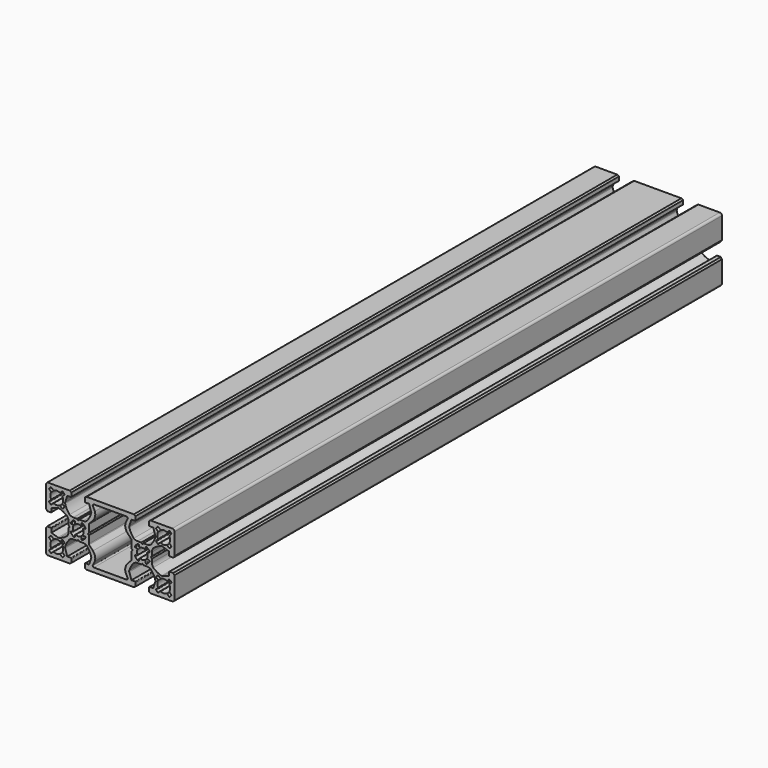
from build123d import *

# Parameters (mm, degrees)
F1_DEPTH = 320


# Not quite as in the source:
# - ends of sketch curves that miss each other by under 0.0002 mm in the source are joined


with BuildPart() as f1:
    # F0 (on Front) → F1 (new body)
    with BuildSketch(Plane.XZ):
        with BuildLine():
            Line((-8.518099, 44.468192), (-7.718099, 43.968192))
            Line((-7.718099, 43.968192), (14.381901, 43.968192))
            Line((14.381901, 43.968192), (15.181901, 44.468192))
            Line((15.181901, 44.468192), (15.181901, 46.168192))
            ThreePointArc((15.181901, 46.168192), (15.0940330344, 46.3803240344), (14.881901, 46.468192))
            Line((14.881901, 46.468192), (13.231901, 46.468192))
            Line((13.231901, 46.468192), (12.244293, 49.519965))
            ThreePointArc((12.244293, 49.519965), (12.1969348994, 49.7784423097), (12.2185454366, 50.0403321225))
            ThreePointArc((12.2185454366, 50.0403321225), (13.0572387483, 52.0781116138), (14.3278880705, 53.8785009374))
            ThreePointArc((14.3278880705, 53.8785009374), (15.1735620055, 54.3169572628), (16.11406, 54.468192))
            Line((16.11406, 54.468192), (17.831901, 54.468192))
            Line((17.831901, 54.468192), (18.331901, 54.968192))
            Line((18.331901, 54.968192), (18.831901, 54.468192))
            Line((18.831901, 54.468192), (20.549742, 54.468192))
            ThreePointArc((20.549742, 54.468192), (21.4902399945, 54.3169572628), (22.335914011, 53.8785010149))
            ThreePointArc((22.335914011, 53.8785010149), (23.6065633179, 52.0781114934), (24.4452563402, 50.0403318114))
            ThreePointArc((24.4452563402, 50.0403318114), (24.4668670953, 49.7784422036), (24.4195087246, 49.5199650891))
            Line((24.4195087246, 49.5199650891), (23.431901, 46.468192))
            Line((23.431901, 46.468192), (21.781901, 46.468192))
            ThreePointArc((21.781901, 46.468192), (21.5697689656, 46.3803240344), (21.481901, 46.168192))
            Line((21.481901, 46.168192), (21.481901, 44.468192))
            Line((21.481901, 44.468192), (22.281901, 43.968192))
            Line((22.281901, 43.968192), (32.331901, 43.968192))
            ThreePointArc((32.331901, 43.968192), (33.0390077812, 44.2610852188), (33.331901, 44.968192))
            Line((33.331901, 44.968192), (33.331901, 55.018192))
            Line((33.331901, 55.018192), (32.831901, 55.818192))
            Line((32.831901, 55.818192), (31.131901, 55.818192))
            ThreePointArc((31.131901, 55.818192), (30.9197689656, 55.7303240344), (30.831901, 55.518192))
            Line((30.831901, 55.518192), (30.831901, 53.868192))
            Line((30.831901, 53.868192), (27.780128, 52.880584))
            ThreePointArc((27.780128, 52.880584), (27.5216507964, 52.8332259047), (27.2597610851, 52.8548363914))
            ThreePointArc((27.2597610851, 52.8548363914), (25.2219810951, 53.6935289083), (23.4215915661, 54.9641785119))
            ThreePointArc((23.4215915661, 54.9641785119), (22.9831357372, 55.8098530055), (22.831901, 56.750351))
            Line((22.831901, 56.750351), (22.831901, 58.468192))
            Line((22.831901, 58.468192), (22.331901, 58.968192))
            Line((22.331901, 58.968192), (22.831901, 59.468192))
            Line((22.831901, 59.468192), (22.831901, 61.186033))
            ThreePointArc((22.831901, 61.186033), (22.9831357372, 62.1265309945), (23.4215919851, 62.972205011))
            ThreePointArc((23.4215919851, 62.972205011), (25.2219813862, 64.2428542517), (27.2597609244, 65.0815472647))
            ThreePointArc((27.2597609244, 65.0815472647), (27.5216506903, 65.1031581006), (27.7801279109, 65.0557997246))
            Line((27.7801279109, 65.0557997246), (30.831901, 64.068192))
            Line((30.831901, 64.068192), (30.831901, 62.418192))
            ThreePointArc((30.831901, 62.418192), (30.9197689656, 62.2060599656), (31.131901, 62.118192))
            Line((31.131901, 62.118192), (32.831901, 62.118192))
            Line((32.831901, 62.118192), (33.331901, 62.918192))
            Line((33.331901, 62.918192), (33.331901, 72.968192))
            ThreePointArc((33.331901, 72.968192), (33.0390077812, 73.6752987812), (32.331901, 73.968192))
            Line((32.331901, 73.968192), (22.281901, 73.968192))
            Line((22.281901, 73.968192), (21.481901, 73.468192))
            Line((21.481901, 73.468192), (21.481901, 71.768192))
            ThreePointArc((21.481901, 71.768192), (21.5697689656, 71.5560599656), (21.781901, 71.468192))
            Line((21.781901, 71.468192), (23.431901, 71.468192))
            Line((23.431901, 71.468192), (24.419509, 68.416418))
            ThreePointArc((24.419509, 68.416418), (24.4668671188, 68.1579413212), (24.4452566086, 67.8960520851))
            ThreePointArc((24.4452566086, 67.8960520851), (23.6065633179, 65.8582725066), (22.3359139295, 64.0578830626))
            ThreePointArc((22.3359139295, 64.0578830626), (21.4902399945, 63.6194267372), (20.549742, 63.468192))
            Line((20.549742, 63.468192), (18.831901, 63.468192))
            Line((18.831901, 63.468192), (18.331901, 62.968192))
            Line((18.331901, 62.968192), (17.831901, 63.468192))
            Line((17.831901, 63.468192), (16.11406, 63.468192))
            ThreePointArc((16.11406, 63.468192), (15.1735620055, 63.6194267372), (14.327887989, 64.0578829851))
            ThreePointArc((14.327887989, 64.0578829851), (13.0572387483, 65.8582723862), (12.2185457353, 67.8960519244))
            ThreePointArc((12.2185457353, 67.8960519244), (12.1969348759, 68.1579412151), (12.2442929825, 68.4164180057))
            Line((12.2442929825, 68.4164180057), (13.231901, 71.468192))
            Line((13.231901, 71.468192), (14.881901, 71.468192))
            ThreePointArc((14.881901, 71.468192), (15.0940330344, 71.5560599656), (15.181901, 71.768192))
            Line((15.181901, 71.768192), (15.181901, 73.468192))
            Line((15.181901, 73.468192), (14.381901, 73.968192))
            Line((14.381901, 73.968192), (-7.718099, 73.968192))
            Line((-7.718099, 73.968192), (-8.518099, 73.468192))
            Line((-8.518099, 73.468192), (-8.518099, 71.768192))
            ThreePointArc((-8.518099, 71.768192), (-8.4302310344, 71.5560599656), (-8.218099, 71.468192))
            Line((-8.218099, 71.468192), (-6.568099, 71.468192))
            Line((-6.568099, 71.468192), (-5.580491, 68.416418))
            ThreePointArc((-5.580491, 68.416418), (-5.5331328812, 68.1579413212), (-5.5547433914, 67.8960520851))
            ThreePointArc((-5.5547433914, 67.8960520851), (-6.3934366821, 65.8582725066), (-7.6640860705, 64.0578830626))
            ThreePointArc((-7.6640860705, 64.0578830626), (-8.5097600055, 63.6194267372), (-9.450258, 63.468192))
            Line((-9.450258, 63.468192), (-11.168099, 63.468192))
            Line((-11.168099, 63.468192), (-11.668099, 62.968192))
            Line((-11.668099, 62.968192), (-12.168099, 63.468192))
            Line((-12.168099, 63.468192), (-13.88594, 63.468192))
            ThreePointArc((-13.88594, 63.468192), (-14.8264379945, 63.6194267372), (-15.672112011, 64.0578829851))
            ThreePointArc((-15.672112011, 64.0578829851), (-16.9427612517, 65.8582723862), (-17.7814542647, 67.8960519244))
            ThreePointArc((-17.7814542647, 67.8960519244), (-17.8030651241, 68.1579412151), (-17.7557070175, 68.4164180057))
            Line((-17.7557070175, 68.4164180057), (-16.768099, 71.468192))
            Line((-16.768099, 71.468192), (-15.118099, 71.468192))
            ThreePointArc((-15.118099, 71.468192), (-14.9059669656, 71.5560599656), (-14.818099, 71.768192))
            Line((-14.818099, 71.768192), (-14.818099, 73.468192))
            Line((-14.818099, 73.468192), (-15.618099, 73.968192))
            Line((-15.618099, 73.968192), (-25.668099, 73.968192))
            ThreePointArc((-25.668099, 73.968192), (-26.3752057812, 73.6752987812), (-26.668099, 72.968192))
            Line((-26.668099, 72.968192), (-26.668099, 62.918192))
            Line((-26.668099, 62.918192), (-26.168099, 62.118192))
            Line((-26.168099, 62.118192), (-24.468099, 62.118192))
            ThreePointArc((-24.468099, 62.118192), (-24.2559669656, 62.2060599656), (-24.168099, 62.418192))
            Line((-24.168099, 62.418192), (-24.168099, 64.068192))
            Line((-24.168099, 64.068192), (-21.116325, 65.0558))
            ThreePointArc((-21.116325, 65.0558), (-20.8578482151, 65.1031581241), (-20.5959588775, 65.0815475634))
            ThreePointArc((-20.5959588775, 65.0815475634), (-18.5581793862, 64.2428542517), (-16.7577900626, 62.9722049295))
            ThreePointArc((-16.7577900626, 62.9722049295), (-16.3193337372, 62.1265309945), (-16.168099, 61.186033))
            Line((-16.168099, 61.186033), (-16.168099, 59.468192))
            Line((-16.168099, 59.468192), (-15.668099, 58.968192))
            Line((-15.668099, 58.968192), (-16.168099, 58.468192))
            Line((-16.168099, 58.468192), (-16.168099, 56.750351))
            ThreePointArc((-16.168099, 56.750351), (-16.3193337372, 55.8098530055), (-16.7577899851, 54.964178989))
            ThreePointArc((-16.7577899851, 54.964178989), (-18.5581790951, 53.6935289083), (-20.5959589244, 52.8548357353))
            ThreePointArc((-20.5959589244, 52.8548357353), (-20.8578483212, 52.8332258812), (-21.1163250057, 52.8805839825))
            Line((-21.1163250057, 52.8805839825), (-24.168099, 53.868192))
            Line((-24.168099, 53.868192), (-24.168099, 55.518192))
            ThreePointArc((-24.168099, 55.518192), (-24.2559669656, 55.7303240344), (-24.468099, 55.818192))
            Line((-24.468099, 55.818192), (-26.168099, 55.818192))
            Line((-26.168099, 55.818192), (-26.668099, 55.018192))
            Line((-26.668099, 55.018192), (-26.668099, 44.968192))
            ThreePointArc((-26.668099, 44.968192), (-26.3752057812, 44.2610852188), (-25.668099, 43.968192))
            Line((-25.668099, 43.968192), (-15.618099, 43.968192))
            Line((-15.618099, 43.968192), (-14.818099, 44.468192))
            Line((-14.818099, 44.468192), (-14.818099, 46.168192))
            ThreePointArc((-14.818099, 46.168192), (-14.9059669656, 46.3803240344), (-15.118099, 46.468192))
            Line((-15.118099, 46.468192), (-16.768099, 46.468192))
            Line((-16.768099, 46.468192), (-17.755707, 49.519965))
            ThreePointArc((-17.755707, 49.519965), (-17.8030651006, 49.7784423097), (-17.7814545634, 50.0403321225))
            ThreePointArc((-17.7814545634, 50.0403321225), (-16.9427612517, 52.0781116138), (-15.6721119295, 53.8785009374))
            ThreePointArc((-15.6721119295, 53.8785009374), (-14.8264379945, 54.3169572628), (-13.88594, 54.468192))
            Line((-13.88594, 54.468192), (-12.168099, 54.468192))
            Line((-12.168099, 54.468192), (-11.668099, 54.968192))
            Line((-11.668099, 54.968192), (-11.168099, 54.468192))
            Line((-11.168099, 54.468192), (-9.450258, 54.468192))
            ThreePointArc((-9.450258, 54.468192), (-8.5097600055, 54.3169572628), (-7.664085989, 53.8785010149))
            ThreePointArc((-7.664085989, 53.8785010149), (-6.3934366821, 52.0781114934), (-5.5547436598, 50.0403318114))
            ThreePointArc((-5.5547436598, 50.0403318114), (-5.5331329047, 49.7784422036), (-5.5804912754, 49.5199650891))
            Line((-5.5804912754, 49.5199650891), (-6.568099, 46.468192))
            Line((-6.568099, 46.468192), (-8.218099, 46.468192))
            ThreePointArc((-8.218099, 46.468192), (-8.4302310344, 46.3803240344), (-8.518099, 46.168192))
            Line((-8.518099, 46.168192), (-8.518099, 44.468192))
        make_face()
        with BuildLine():
            ThreePointArc((-18.9249375337, 50.6494775338), (-19.0088693342, 50.4856986912), (-18.9813826295, 50.3037301843))
            ThreePointArc((-18.9813826295, 50.3037301843), (-18.6673190091, 48.9676456686), (-18.9811745628, 47.6315122799))
            ThreePointArc((-18.9811745628, 47.6315122799), (-19.0086328238, 47.4495393277), (-18.9246755337, 47.2857734662))
            Line((-18.9246755337, 47.2857734662), (-18.184047, 46.545261))
            ThreePointArc((-18.184047, 46.545261), (-18.0965953169, 46.3492303869), (-18.1625078476, 46.1449478773))
            ThreePointArc((-18.1625078476, 46.1449478773), (-18.4850900769, 45.7856799118), (-18.8443080142, 45.4630420176))
            ThreePointArc((-18.8443080142, 45.4630420176), (-19.0485799503, 45.3970967683), (-19.2446245337, 45.4845174662))
            Line((-19.2446245337, 45.4845174662), (-19.985253, 46.225031))
            ThreePointArc((-19.985253, 46.225031), (-20.1490316578, 46.3089623911), (-20.3309998157, 46.2814756295))
            ThreePointArc((-20.3309998157, 46.2814756295), (-21.6670844361, 45.9674120092), (-23.0032179184, 46.281267164))
            ThreePointArc((-23.0032179184, 46.281267164), (-23.1851910212, 46.3087257668), (-23.3489570337, 46.2247680337))
            Line((-23.3489570337, 46.2247680337), (-24.08947, 45.48414))
            ThreePointArc((-24.08947, 45.48414), (-24.2855006131, 45.3966883169), (-24.4897831227, 45.4626008476))
            ThreePointArc((-24.4897831227, 45.4626008476), (-24.8490510882, 45.7851830769), (-25.1716889824, 46.1444010142))
            ThreePointArc((-25.1716889824, 46.1444010142), (-25.2376332338, 46.3486729105), (-25.1502130337, 46.5447170337))
            Line((-25.1502130337, 46.5447170337), (-24.4097, 47.285346))
            ThreePointArc((-24.4097, 47.285346), (-24.3257676299, 47.4491245287), (-24.3532545689, 47.6310932145))
            ThreePointArc((-24.3532545689, 47.6310932145), (-24.6673189908, 48.9671776587), (-24.3534636377, 50.3033113171))
            ThreePointArc((-24.3534636377, 50.3033113171), (-24.3260052121, 50.485283892), (-24.4099624662, 50.6490495337))
            Line((-24.4099624662, 50.6490495337), (-25.150591, 51.389563))
            ThreePointArc((-25.150591, 51.389563), (-25.2380417021, 51.5855939661), (-25.1721291524, 51.7898761227))
            ThreePointArc((-25.1721291524, 51.7898761227), (-24.8495477014, 52.14914431), (-24.4903299858, 52.4717819824))
            ThreePointArc((-24.4903299858, 52.4717819824), (-24.2860577364, 52.5377262149), (-24.0900134662, 52.4503055337))
            Line((-24.0900134662, 52.4503055337), (-23.349385, 51.709793))
            ThreePointArc((-23.349385, 51.709793), (-23.1856058203, 51.6258606869), (-23.0036367855, 51.6533475689))
            ThreePointArc((-23.0036367855, 51.6533475689), (-21.6675524459, 51.9674119909), (-20.3314188812, 51.653556239))
            ThreePointArc((-20.3314188812, 51.653556239), (-20.1494464569, 51.626098155), (-19.9856809662, 51.7100549662))
            Line((-19.9856809662, 51.7100549662), (-19.245168, 52.450684))
            ThreePointArc((-19.245168, 52.450684), (-19.0491370339, 52.5381347021), (-18.8448548773, 52.4722221524))
            ThreePointArc((-18.8448548773, 52.4722221524), (-18.48558669, 52.1496407014), (-18.1629490176, 51.7904229858))
            ThreePointArc((-18.1629490176, 51.7904229858), (-18.0970037873, 51.5861506966), (-18.1844249662, 51.3901059662))
            Line((-18.1844249662, 51.3901059662), (-18.9249375337, 50.6494775338))
        make_face(mode=Mode.SUBTRACT)
        with BuildLine():
            ThreePointArc((-8.2257142903, 61.0021958284), (-8.2112073588, 60.7246798967), (-8.4307570125, 60.5543170693))
            Line((-8.4307570125, 60.5543170693), (-9.171691, 60.420746))
            ThreePointArc((-9.171691, 60.420746), (-9.3841243726, 60.2648808555), (-9.3916412479, 60.0015078875))
            ThreePointArc((-9.3916412479, 60.0015078875), (-9.168099, 58.968192), (-9.391641543, 57.9348762465))
            ThreePointArc((-9.391641543, 57.9348762465), (-9.3841245841, 57.6715025477), (-9.171690956, 57.5156372439))
            Line((-9.171690956, 57.5156372439), (-8.430757, 57.382067))
            ThreePointArc((-8.430757, 57.382067), (-8.2112073588, 57.2117041033), (-8.2257142903, 56.9341881716))
            ThreePointArc((-8.2257142903, 56.9341881716), (-8.8408418753, 56.1409348753), (-9.6340952702, 55.5258074572))
            ThreePointArc((-9.6340952702, 55.5258074572), (-9.9116111033, 55.5113003588), (-10.0819739307, 55.7308500125))
            Line((-10.0819739307, 55.7308500125), (-10.215544, 56.471784))
            ThreePointArc((-10.215544, 56.471784), (-10.3714095477, 56.6842175841), (-10.6347829417, 56.6917338716))
            ThreePointArc((-10.6347829417, 56.6917338716), (-11.668099, 56.468192), (-12.7014147535, 56.691734543))
            ThreePointArc((-12.7014147535, 56.691734543), (-12.9647878555, 56.6842173726), (-13.1206527561, 56.471783956))
            Line((-13.1206527561, 56.471783956), (-13.254224, 55.73085))
            ThreePointArc((-13.254224, 55.73085), (-13.4245868967, 55.5113003588), (-13.7021028284, 55.5258072903))
            ThreePointArc((-13.7021028284, 55.5258072903), (-14.4953559449, 56.1409346954), (-15.110483284, 56.9341878322))
            ThreePointArc((-15.110483284, 56.9341878322), (-15.1249907471, 57.211703872), (-14.9054409875, 57.3820669307))
            Line((-14.9054409875, 57.3820669307), (-14.164507, 57.515637))
            ThreePointArc((-14.164507, 57.515637), (-13.9520726445, 57.671502112), (-13.9445561284, 57.9348759417))
            ThreePointArc((-13.9445561284, 57.9348759417), (-14.168099, 58.968192), (-13.9445562862, 60.0015081299))
            ThreePointArc((-13.9445562862, 60.0015081299), (-13.9520728561, 60.2648812912), (-14.1645070125, 60.4207459307))
            Line((-14.1645070125, 60.4207459307), (-14.905441, 60.554317))
            ThreePointArc((-14.905441, 60.554317), (-15.1249907471, 60.724680128), (-15.1104834508, 61.0021962664))
            ThreePointArc((-15.1104834508, 61.0021962664), (-14.4953561247, 61.7954491247), (-13.7021031678, 62.410576284))
            ThreePointArc((-13.7021031678, 62.410576284), (-13.424587128, 62.4250837471), (-13.2542240693, 62.2055339875))
            Line((-13.2542240693, 62.2055339875), (-13.120653, 61.4646))
            ThreePointArc((-13.120653, 61.4646), (-12.9647882912, 61.2521658561), (-12.7014148875, 61.2446487521))
            ThreePointArc((-12.7014148875, 61.2446487521), (-11.668099, 61.468192), (-10.6347828701, 61.2446492862))
            ThreePointArc((-10.6347828701, 61.2446492862), (-10.371409112, 61.2521656445), (-10.2155440693, 61.4646000125))
            Line((-10.2155440693, 61.4646000125), (-10.081974, 62.205534))
            ThreePointArc((-10.081974, 62.205534), (-9.911610872, 62.4250837471), (-9.6340947336, 62.4105764508))
            ThreePointArc((-9.6340947336, 62.4105764508), (-8.8408416954, 61.7954489449), (-8.2257142903, 61.0021958284))
        make_face(mode=Mode.SUBTRACT)
        with BuildLine():
            ThreePointArc((25.642636761, 47.6315118812), (25.3287810091, 48.9676454459), (25.6428447006, 50.303730149))
            ThreePointArc((25.6428447006, 50.303730149), (25.6703323131, 50.4856988203), (25.5864000338, 50.6494780338))
            Line((25.5864000338, 50.6494780338), (24.845887, 51.390106))
            ThreePointArc((24.845887, 51.390106), (24.7584667851, 51.5861507364), (24.8244113336, 51.7904227313))
            ThreePointArc((24.8244113336, 51.7904227313), (25.14704869, 52.1496407014), (25.5063167329, 52.4722223317))
            ThreePointArc((25.5063167329, 52.4722223317), (25.710599292, 52.538134742), (25.9066300338, 52.4506840338))
            Line((25.9066300338, 52.4506840338), (26.647143, 51.710055))
            ThreePointArc((26.647143, 51.710055), (26.810909108, 51.6260982121), (26.9928817727, 51.6535564571))
            ThreePointArc((26.9928817727, 51.6535564571), (28.3290153413, 51.9674119908), (29.6650999506, 51.6533479006))
            ThreePointArc((29.6650999506, 51.6533479006), (29.8470684713, 51.6258606299), (30.0108475337, 51.7097924662))
            Line((30.0108475337, 51.7097924662), (30.751476, 52.450306))
            ThreePointArc((30.751476, 52.450306), (30.9475200895, 52.5377262338), (31.1517917313, 52.4717816664))
            ThreePointArc((31.1517917313, 52.4717816664), (31.5110099231, 52.1491440882), (31.8335917251, 51.7898757786))
            ThreePointArc((31.8335917251, 51.7898757786), (31.8995046831, 51.5855936131), (31.8120530337, 51.3895629663))
            Line((31.8120530337, 51.3895629663), (31.071425, 50.64905))
            ThreePointArc((31.071425, 50.64905), (30.9874672332, 50.4852840212), (31.0149256554, 50.3033108286))
            ThreePointArc((31.0149256554, 50.3033108286), (31.3287809908, 48.9671774361), (31.0147169006, 47.6310930494))
            ThreePointArc((31.0147169006, 47.6310930494), (30.9872306089, 47.4491246578), (31.0711619663, 47.2853459663))
            Line((31.0711619663, 47.2853459663), (31.811675, 46.544717))
            ThreePointArc((31.811675, 46.544717), (31.8990962317, 46.3486729503), (31.8331512729, 46.1444007802))
            ThreePointArc((31.8331512729, 46.1444007802), (31.5105130882, 45.7851830769), (31.1512447786, 45.4626012749))
            ThreePointArc((31.1512447786, 45.4626012749), (30.9469626131, 45.3966883169), (30.7509319663, 45.4841399663))
            Line((30.7509319663, 45.4841399663), (30.010419, 46.224768))
            ThreePointArc((30.010419, 46.224768), (29.8466536723, 46.3087258238), (29.6646808286, 46.2812673446))
            ThreePointArc((29.6646808286, 46.2812673446), (28.3285473314, 45.9674120091), (26.992462851, 46.2814757006))
            ThreePointArc((26.992462851, 46.2814757006), (26.8104943088, 46.3089623342), (26.6467154662, 46.2250305337))
            Line((26.6467154662, 46.2250305337), (25.906087, 45.484518))
            ThreePointArc((25.906087, 45.484518), (25.7100426922, 45.3970968081), (25.5057703866, 45.4630412386))
            ThreePointArc((25.5057703866, 45.4630412386), (25.1465525739, 45.7856794147), (24.8239706683, 46.1449477329))
            ThreePointArc((24.8239706683, 46.1449477329), (24.7580582979, 46.3492300339), (24.8455094662, 46.5452605337))
            Line((24.8455094662, 46.5452605337), (25.586138, 47.285774))
            ThreePointArc((25.586138, 47.285774), (25.670094845, 47.4495394569), (25.642636761, 47.6315118812))
        make_face(mode=Mode.SUBTRACT)
        with BuildLine():
            ThreePointArc((21.7742857097, 61.0021958284), (21.7887926412, 60.7246798967), (21.5692429875, 60.5543170693))
            Line((21.5692429875, 60.5543170693), (20.828309, 60.420746))
            ThreePointArc((20.828309, 60.420746), (20.6158756274, 60.2648808555), (20.6083587521, 60.0015078875))
            ThreePointArc((20.6083587521, 60.0015078875), (20.831901, 58.968192), (20.608358457, 57.9348762465))
            ThreePointArc((20.608358457, 57.9348762465), (20.6158754159, 57.6715025477), (20.828309044, 57.5156372439))
            Line((20.828309044, 57.5156372439), (21.569243, 57.382067))
            ThreePointArc((21.569243, 57.382067), (21.7887926412, 57.2117041033), (21.7742857097, 56.9341881716))
            ThreePointArc((21.7742857097, 56.9341881716), (21.1591581247, 56.1409348753), (20.3659047298, 55.5258074572))
            ThreePointArc((20.3659047298, 55.5258074572), (20.0883888967, 55.5113003588), (19.9180260693, 55.7308500125))
            Line((19.9180260693, 55.7308500125), (19.784456, 56.471784))
            ThreePointArc((19.784456, 56.471784), (19.6285904523, 56.6842175841), (19.3652170583, 56.6917338716))
            ThreePointArc((19.3652170583, 56.6917338716), (18.331901, 56.468192), (17.2985852465, 56.691734543))
            ThreePointArc((17.2985852465, 56.691734543), (17.0352121445, 56.6842173726), (16.8793472439, 56.471783956))
            Line((16.8793472439, 56.471783956), (16.745776, 55.73085))
            ThreePointArc((16.745776, 55.73085), (16.5754131033, 55.5113003588), (16.2978971716, 55.5258072903))
            ThreePointArc((16.2978971716, 55.5258072903), (15.5046440551, 56.1409346954), (14.889516716, 56.9341878322))
            ThreePointArc((14.889516716, 56.9341878322), (14.8750092529, 57.211703872), (15.0945590125, 57.3820669307))
            Line((15.0945590125, 57.3820669307), (15.835493, 57.515637))
            ThreePointArc((15.835493, 57.515637), (16.0479273555, 57.671502112), (16.0554438716, 57.9348759417))
            ThreePointArc((16.0554438716, 57.9348759417), (15.831901, 58.968192), (16.0554437138, 60.0015081299))
            ThreePointArc((16.0554437138, 60.0015081299), (16.0479271439, 60.2648812912), (15.8354929875, 60.4207459307))
            Line((15.8354929875, 60.4207459307), (15.094559, 60.554317))
            ThreePointArc((15.094559, 60.554317), (14.8750092529, 60.724680128), (14.8895165492, 61.0021962664))
            ThreePointArc((14.8895165492, 61.0021962664), (15.5046438753, 61.7954491247), (16.2978968322, 62.410576284))
            ThreePointArc((16.2978968322, 62.410576284), (16.575412872, 62.4250837471), (16.7457759307, 62.2055339875))
            Line((16.7457759307, 62.2055339875), (16.879347, 61.4646))
            ThreePointArc((16.879347, 61.4646), (17.0352117088, 61.2521658561), (17.2985851125, 61.2446487521))
            ThreePointArc((17.2985851125, 61.2446487521), (18.331901, 61.468192), (19.3652171299, 61.2446492862))
            ThreePointArc((19.3652171299, 61.2446492862), (19.628590888, 61.2521656445), (19.7844559307, 61.4646000125))
            Line((19.7844559307, 61.4646000125), (19.918026, 62.205534))
            ThreePointArc((19.918026, 62.205534), (20.088389128, 62.4250837471), (20.3659052664, 62.4105764508))
            ThreePointArc((20.3659052664, 62.4105764508), (21.1591583046, 61.7954489449), (21.7742857097, 61.0021958284))
        make_face(mode=Mode.SUBTRACT)
        with BuildLine():
            ThreePointArc((-18.9820587227, 70.304301138), (-18.668099, 68.968192), (-18.9820587227, 67.632082862))
            ThreePointArc((-18.9820587227, 67.632082862), (-19.0095315799, 67.4501123181), (-18.9255870344, 67.2863399656))
            Line((-18.9255870344, 67.2863399656), (-18.185016, 66.545769))
            ThreePointArc((-18.185016, 66.545769), (-18.0975800386, 66.3497316109), (-18.1635086374, 66.1454545134))
            ThreePointArc((-18.1635086374, 66.1454545134), (-18.4861184847, 65.7862114847), (-18.8453615502, 65.4636016831))
            ThreePointArc((-18.8453615502, 65.4636016831), (-19.0496386109, 65.3976730386), (-19.2456760344, 65.4851089656))
            Line((-19.2456760344, 65.4851089656), (-19.986247, 66.22568))
            ThreePointArc((-19.986247, 66.22568), (-20.1500194473, 66.309623601), (-20.3319895952, 66.2821511862))
            ThreePointArc((-20.3319895952, 66.2821511862), (-21.668099, 65.968192), (-23.004208138, 66.2821517227))
            ThreePointArc((-23.004208138, 66.2821517227), (-23.1861785527, 66.309623601), (-23.3499505344, 66.2256795344))
            Line((-23.3499505344, 66.2256795344), (-24.090522, 65.485109))
            ThreePointArc((-24.090522, 65.485109), (-24.2865590002, 65.3976730595), (-24.4908358801, 65.4636011489))
            ThreePointArc((-24.4908358801, 65.4636011489), (-24.8500790182, 65.7862109875), (-25.1726889234, 66.1454540617))
            ThreePointArc((-25.1726889234, 66.1454540617), (-25.2386179782, 66.3497312978), (-25.1511820344, 66.5457690344))
            Line((-25.1511820344, 66.5457690344), (-24.410611, 67.28634))
            ThreePointArc((-24.410611, 67.28634), (-24.3266664201, 67.4501123181), (-24.3541390121, 67.632082994))
            ThreePointArc((-24.3541390121, 67.632082994), (-24.668099, 68.968192), (-24.3541392773, 70.304301138))
            ThreePointArc((-24.3541392773, 70.304301138), (-24.3266664201, 70.4862716819), (-24.4106109656, 70.6500440344))
            Line((-24.4106109656, 70.6500440344), (-25.151182, 71.390615))
            ThreePointArc((-25.151182, 71.390615), (-25.2386179573, 71.5866523134), (-25.1726894576, 71.7909293686))
            ThreePointArc((-25.1726894576, 71.7909293686), (-24.8500795153, 72.1501725153), (-24.4908363318, 72.472782412))
            ThreePointArc((-24.4908363318, 72.472782412), (-24.2865593134, 72.5387109573), (-24.0905219656, 72.4512750344))
            Line((-24.0905219656, 72.4512750344), (-23.349951, 71.710704))
            ThreePointArc((-23.349951, 71.710704), (-23.1861786819, 71.6267594201), (-23.004208006, 71.6542320121))
            ThreePointArc((-23.004208006, 71.6542320121), (-21.668099, 71.968192), (-20.331989862, 71.6542322773))
            ThreePointArc((-20.331989862, 71.6542322773), (-20.1500193181, 71.6267594201), (-19.9862469656, 71.7107039656))
            Line((-19.9862469656, 71.7107039656), (-19.245676, 72.451275))
            ThreePointArc((-19.245676, 72.451275), (-19.0496382978, 72.5387109782), (-18.8453610249, 72.4727819691))
            ThreePointArc((-18.8453610249, 72.4727819691), (-18.4861179875, 72.1501720182), (-18.1635081946, 71.7909288433))
            ThreePointArc((-18.1635081946, 71.7909288433), (-18.0975800595, 71.5866520002), (-18.1850159656, 71.3906149656))
            Line((-18.1850159656, 71.3906149656), (-18.925587, 70.650044))
            ThreePointArc((-18.925587, 70.650044), (-19.0095315799, 70.4862716819), (-18.9820587227, 70.304301138))
        make_face(mode=Mode.SUBTRACT)
        with BuildLine():
            ThreePointArc((10.5347299963, 69.2257660012), (10.4246817794, 67.1116653149), (11.4090291392, 65.23747413))
            Line((11.4090291392, 65.23747413), (13.19726, 63.32341))
            ThreePointArc((13.19726, 63.32341), (13.2970243325, 63.1655373964), (13.331901, 62.98207))
            Line((13.331901, 62.98207), (13.331901, 59.468192))
            Line((13.331901, 59.468192), (13.831901, 58.968192))
            Line((13.831901, 58.968192), (13.331901, 58.468192))
            Line((13.331901, 58.468192), (13.331901, 54.954314))
            ThreePointArc((13.331901, 54.954314), (13.2970243325, 54.7708466036), (13.1972598579, 54.6129741328))
            Line((13.1972598579, 54.6129741328), (11.409029, 52.69891))
            ThreePointArc((11.409029, 52.69891), (10.4246816778, 50.8247182215), (10.5347302947, 48.7106170976))
            Line((10.5347302947, 48.7106170976), (11.478698, 46.678868))
            ThreePointArc((11.478698, 46.678868), (11.4467569605, 46.1992476949), (11.025249, 45.968192))
            Line((11.025249, 45.968192), (-4.361447, 45.968192))
            ThreePointArc((-4.361447, 45.968192), (-4.7829550738, 46.1992478725), (-4.8148954846, 46.6788682251))
            Line((-4.8148954846, 46.6788682251), (-3.870928, 48.710617))
            ThreePointArc((-3.870928, 48.710617), (-3.7608796778, 50.8247182215), (-4.7452271392, 52.69890987))
            Line((-4.7452271392, 52.69890987), (-6.533458, 54.612974))
            ThreePointArc((-6.533458, 54.612974), (-6.6332223325, 54.7708466036), (-6.668099, 54.954314))
            Line((-6.668099, 54.954314), (-6.668099, 58.468192))
            Line((-6.668099, 58.468192), (-7.168099, 58.968192))
            Line((-7.168099, 58.968192), (-6.668099, 59.468192))
            Line((-6.668099, 59.468192), (-6.668099, 62.98207))
            ThreePointArc((-6.668099, 62.98207), (-6.6332223325, 63.1655373964), (-6.5334578579, 63.3234098672))
            Line((-6.5334578579, 63.3234098672), (-4.745227, 65.237474))
            ThreePointArc((-4.745227, 65.237474), (-3.7608797794, 67.1116653149), (-3.8709279963, 69.2257660012))
            Line((-3.8709279963, 69.2257660012), (-4.814895, 71.257516))
            ThreePointArc((-4.814895, 71.257516), (-4.7829550738, 71.7371361275), (-4.361447, 71.968192))
            Line((-4.361447, 71.968192), (11.025249, 71.968192))
            ThreePointArc((11.025249, 71.968192), (11.4467569605, 71.7371363051), (11.4786976621, 71.257516157))
            Line((11.4786976621, 71.257516157), (10.5347299963, 69.2257660012))
        make_face(mode=Mode.SUBTRACT)
        with BuildLine():
            ThreePointArc((25.5870490344, 67.2863399656), (25.6709935799, 67.4501123181), (25.6435209879, 67.632082994))
            ThreePointArc((25.6435209879, 67.632082994), (25.329561, 68.968192), (25.6435207227, 70.304301138))
            ThreePointArc((25.6435207227, 70.304301138), (25.6709935799, 70.4862716819), (25.5870490344, 70.6500440344))
            Line((25.5870490344, 70.6500440344), (24.846478, 71.390615))
            ThreePointArc((24.846478, 71.390615), (24.7590420427, 71.5866523134), (24.8249705424, 71.7909293686))
            ThreePointArc((24.8249705424, 71.7909293686), (25.1475804847, 72.1501725153), (25.5068236682, 72.472782412))
            ThreePointArc((25.5068236682, 72.472782412), (25.7111006866, 72.5387109573), (25.9071380344, 72.4512750344))
            Line((25.9071380344, 72.4512750344), (26.647709, 71.710704))
            ThreePointArc((26.647709, 71.710704), (26.8114813181, 71.6267594201), (26.993451994, 71.6542320121))
            ThreePointArc((26.993451994, 71.6542320121), (28.329561, 71.968192), (29.665670138, 71.6542322773))
            ThreePointArc((29.665670138, 71.6542322773), (29.8476406819, 71.6267594201), (30.0114130344, 71.7107039656))
            Line((30.0114130344, 71.7107039656), (30.751984, 72.451275))
            ThreePointArc((30.751984, 72.451275), (30.9480217022, 72.5387109782), (31.1522989751, 72.4727819691))
            ThreePointArc((31.1522989751, 72.4727819691), (31.5115420125, 72.1501720182), (31.8341518054, 71.7909288433))
            ThreePointArc((31.8341518054, 71.7909288433), (31.9000799405, 71.5866520002), (31.8126440344, 71.3906149656))
            Line((31.8126440344, 71.3906149656), (31.072074, 70.650044))
            ThreePointArc((31.072074, 70.650044), (30.9881294201, 70.4862716819), (31.0156020121, 70.304301006))
            ThreePointArc((31.0156020121, 70.304301006), (31.329561, 68.968192), (31.0156014757, 67.6320832608))
            ThreePointArc((31.0156014757, 67.6320832608), (30.9881294201, 67.4501123181), (31.0720739656, 67.2863399656))
            Line((31.0720739656, 67.2863399656), (31.812644, 66.545769))
            ThreePointArc((31.812644, 66.545769), (31.9000799614, 66.3497316109), (31.8341513626, 66.1454545134))
            ThreePointArc((31.8341513626, 66.1454545134), (31.5115415153, 65.7862114847), (31.1522984498, 65.4636016831))
            ThreePointArc((31.1522984498, 65.4636016831), (30.9480213891, 65.3976730386), (30.7519839656, 65.4851089656))
            Line((30.7519839656, 65.4851089656), (30.011413, 66.22568))
            ThreePointArc((30.011413, 66.22568), (29.8476405527, 66.309623601), (29.6656704048, 66.2821511862))
            ThreePointArc((29.6656704048, 66.2821511862), (28.329561, 65.968192), (26.993451862, 66.2821517227))
            ThreePointArc((26.993451862, 66.2821517227), (26.8114814473, 66.309623601), (26.6477094656, 66.2256795344))
            Line((26.6477094656, 66.2256795344), (25.907138, 65.485109))
            ThreePointArc((25.907138, 65.485109), (25.7111009998, 65.3976730595), (25.5068241199, 65.4636011489))
            ThreePointArc((25.5068241199, 65.4636011489), (25.1475809818, 65.7862109875), (24.8249710766, 66.1454540617))
            ThreePointArc((24.8249710766, 66.1454540617), (24.7590420218, 66.3497312978), (24.8464779656, 66.5457690344))
            Line((24.8464779656, 66.5457690344), (25.5870490344, 67.2863399656))
        make_face(mode=Mode.SUBTRACT)
    extrude(amount=F1_DEPTH)


solid = f1.part
